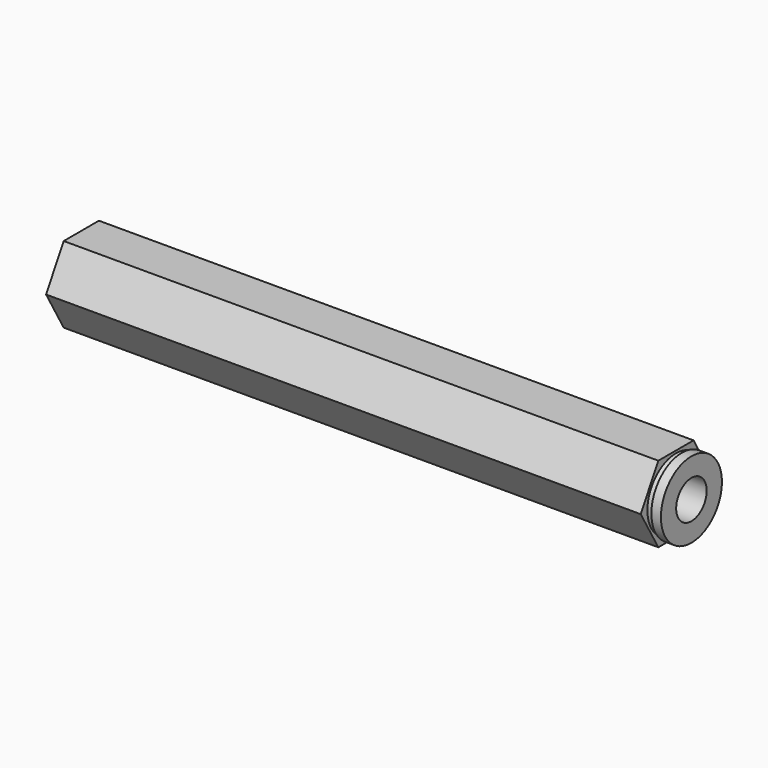
from build123d import *

# Parameters (mm, degrees)
F1_DEPTH = 101.6
F4_R     = 3.175
F5_DEPTH = 101.601


with BuildPart() as f1:
    # F0 (on Right) → F1 (new body)
    with BuildSketch(Plane.YZ):
        Polygon((3.6661742094, 6.35), (-3.6661742094, 6.35), (-7.3323484187, 0), (-3.6661742094, -6.35), (3.6661742094, -6.35), (7.3323484187, 0), align=None)
    extrude(amount=F1_DEPTH)

    # F2 (on Top) → F3 (revolve, cut)
    with BuildSketch(Plane.XY):
        Polygon((100.0125, 6.35), (101.6, 6.35), (101.6, 7.3323484187), (99.0219, 7.3323484187), (99.0219, 5.9436), (100.0125, 5.9436), align=None)
    revolve(axis=Axis((50.8, 0, 0), (1, 0, 0)), mode=Mode.SUBTRACT)

    # F4 (on face) → F5 (cut, through all)
    with BuildSketch(Plane.YZ.offset(101.6)):
        Circle(F4_R)
    extrude(amount=-F5_DEPTH, mode=Mode.SUBTRACT)


solid = f1.part
